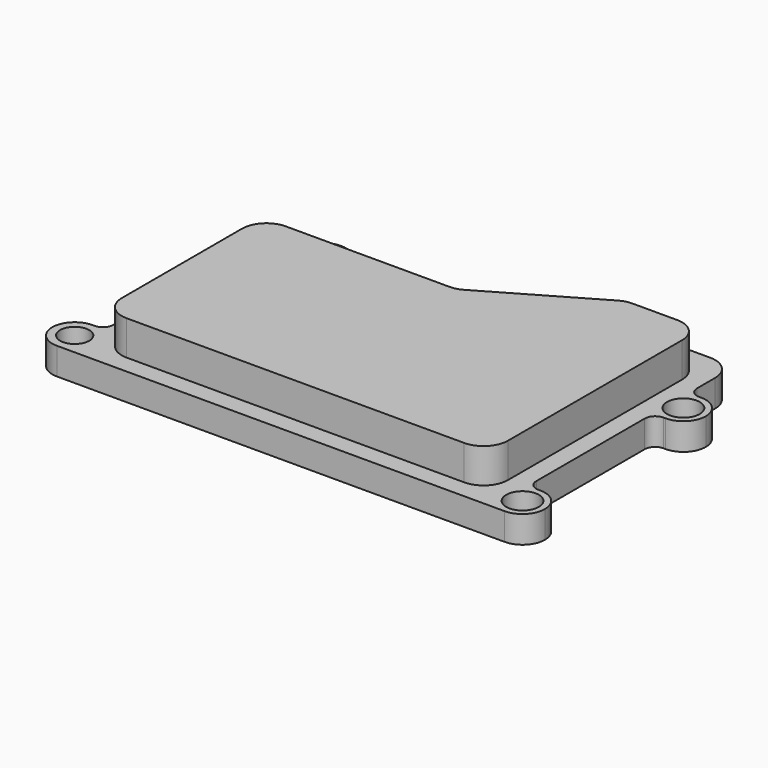
from build123d import *

# Parameters (mm, degrees)
F1_DEPTH  = 7.8
F2_R      = 6.44999
F3_R      = 2.7
F4_DEPTH  = 7.801
F5_R      = 4.2
F5_R_2    = 4.7163688055
F6_DEPTH  = 5.3
F8_DEPTH  = 10
F10_DEPTH = 5.2
F12_DEPTH = 9.8
F13_R     = 5
F14_R     = 7
F15_R     = 3
F16_R     = 3


# Not quite as in the source:
# - a fillet or chamfer is up to 0.001 mm smaller than in the source, because OpenCascade refuses the exact size


with BuildPart() as f1:
    # F0 (on Top) → F1 (new body)
    with BuildSketch(Plane.XY):
        Polygon((0, 68), (0, 12.9), (-10.05, 12.9), (-10.05, 0), (0, 0), (122, 0), (132.05, 0), (132.05, 12.9), (122, 12.9), (122, 58), (132.05, 58), (132.05, 70.9), (122, 70.9), (122, 87.4), (93.5, 87.4), (60, 68), (22.4718242228, 68), (22.4718242228, 78.05), (9.5718242228, 78.05), (9.5718242228, 68), align=None)
    extrude(amount=F1_DEPTH)

    # F2 (radius 6.45 in the source; OpenCascade refuses exactly that, so slightly less here)
    f2_edges = [f1.edges().sort_by_distance(p)[0] for p in [
        (-10.05, 0, 3.9),
        (-10.05, 12.9, 3.9),
        (9.571824, 78.05, 3.9),
        (22.471824, 78.05, 3.9),
        (132.05, 70.9, 3.9),
        (132.05, 58, 3.9),
        (132.05, 12.9, 3.9),
        (132.05, 0, 3.9),
    ]]
    fillet(f2_edges, radius=F2_R)

    # F3 (on face) → F4 (cut, through all)
    with BuildSketch(Plane.XY.offset(7.8)):
        with Locations((-3.6, 6.45)):
            Circle(F3_R)
        with Locations((16.0218242228, 71.6)):
            Circle(F3_R)
        with Locations((125.6, 64.45)):
            Circle(F3_R)
        with Locations((125.6, 6.45)):
            Circle(F3_R)
    extrude(amount=-F4_DEPTH, mode=Mode.SUBTRACT)

    # F5 (on face) → F6 (cut)
    with BuildSketch(Plane.XY.offset(7.8)):
        with Locations((-3.6, 6.45)):
            Circle(F5_R)
        with Locations((16.0218242228, 71.6)):
            Circle(F5_R)
        with Locations((125.6, 64.45)):
            Circle(F5_R_2)
        with Locations((125.6, 6.45)):
            Circle(F5_R_2)
    extrude(amount=-F6_DEPTH, mode=Mode.SUBTRACT)

    # F7 (on face) → F8 (join)
    with BuildSketch(Plane.XY.offset(7.8)):
        Polygon((5.3, 62.7), (5.3, 5.3), (116.7, 5.3), (116.7, 82.1), (94.9238653477, 82.1), (61.4238653477, 62.7), align=None)
    extrude(amount=F8_DEPTH)

    # F9 (on face) → F10 (cut)
    with BuildSketch(Plane(origin=(0, 0, 0), x_dir=(1, 0, 0), z_dir=(0, 0, -1))):
        Polygon((94.0910384462, -85.2), (119.8, -85.2), (119.8, -2.2), (2.2, -2.2), (2.2, -65.8), (60.5910384462, -65.8), align=None)
    extrude(amount=-F10_DEPTH, mode=Mode.SUBTRACT)

    # F11 (on face) → F12 (cut)
    with BuildSketch(Plane(origin=(0, 0, 5.2), x_dir=(1, 0, 0), z_dir=(0, 0, -1))):
        Polygon((114.5, -7.5), (7.5, -7.5), (7.5, -60.5), (62.0149037939, -60.5), (95.5149037939, -79.9), (114.5, -79.9), align=None)
    extrude(amount=-F12_DEPTH, mode=Mode.SUBTRACT)

    # F13
    f13_edges = [f1.edges().sort_by_distance(p)[0] for p in [
        (114.5, 79.9, 10.1),
        (119.8, 85.2, 2.6),
        (7.5, 60.5, 10.1),
        (2.2, 65.8, 2.6),
        (114.5, 7.5, 10.1),
        (7.5, 7.5, 10.1),
        (95.514904, 79.9, 10.1),
        (62.014904, 60.5, 10.1),
        (60.591038, 65.8, 2.6),
        (94.091038, 85.2, 2.6),
    ]]
    fillet(f13_edges, radius=F13_R)

    # F14
    f14_edges = [f1.edges().sort_by_distance(p)[0] for p in [
        (122, 87.4, 3.9),
        (93.5, 87.4, 3.9),
        (60, 68, 3.9),
        (61.423865, 62.7, 12.8),
        (94.923865, 82.1, 12.8),
        (116.7, 82.1, 12.8),
        (116.7, 5.3, 12.8),
        (5.3, 5.3, 12.8),
        (5.3, 62.7, 12.8),
        (0, 68, 3.9),
    ]]
    fillet(f14_edges, radius=F14_R)

    # F15
    f15_edges = [f1.edges().sort_by_distance(p)[0] for p in [
        (119.8, 2.2, 2.6),
        (2.2, 2.2, 2.6),
    ]]
    fillet(f15_edges, radius=F15_R)

    # F16
    f16_edges = [f1.edges().sort_by_distance(p)[0] for p in [
        (0, 12.9, 3.9),
        (9.571824, 68, 3.9),
        (22.471824, 68, 3.9),
        (122, 70.9, 3.9),
        (122, 58, 3.9),
        (122, 12.9, 3.9),
    ]]
    fillet(f16_edges, radius=F16_R)


solid = f1.part
